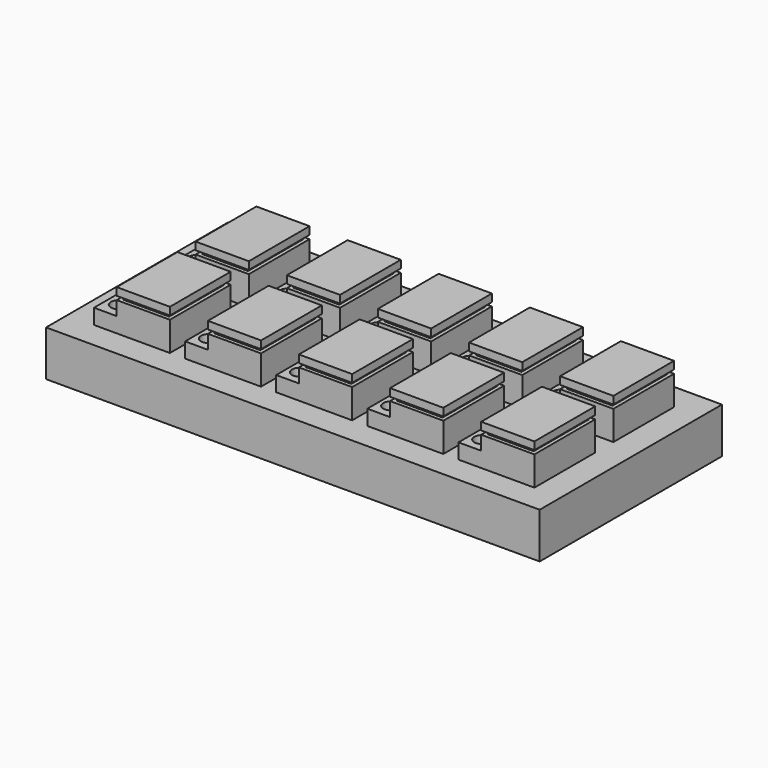
from build123d import *

# Parameters (mm, degrees)
F0_W           = 103.1875
F0_H           = 47.625
F1_DEPTH       = 9.525
F2_W           = 15.875
F2_H           = 15.875
F3_DEPTH       = 3.175
F4_W           = 11.1267840786
F4_H           = 15.875
F5_DEPTH       = 5.334
F6_W           = 11.1309718871
F6_H           = 15.875
F7_DEPTH       = 5.334
F8_W           = 11.1265123679
F8_H           = 15.875
F9_DEPTH       = 5.334
F10_W          = 11.1239126975
F10_H          = 15.875
F11_DEPTH      = 5.334
F12_W          = 11.1350612026
F12_H          = 15.875
F13_DEPTH      = 5.334
F14_W          = 11.1336731828
F14_H          = 15.875
F15_DEPTH      = 5.334
F16_W          = 11.1136997504
F16_H          = 15.875
F17_DEPTH      = 5.334
F18_W          = 11.1152978999
F18_H          = 15.875
F19_DEPTH      = 5.334
F20_W          = 11.1280665679
F20_H          = 15.875
F21_DEPTH      = 5.334
F22_W          = 11.1295790357
F22_H          = 15.875
F23_DEPTH      = 5.334
F24_W          = 11.1267840786
F24_H          = 0.7874
F25_DEPTH      = 0.7874
F26_W          = 15.0876
F26_H          = 0.7874
F27_DEPTH      = 0.7874
F28_W          = 10.3393840786
F28_H          = 0.7874
F29_DEPTH      = 0.7874
F30_W          = 14.3002
F30_H          = 0.7874
F31_DEPTH      = 0.7874
F32_W          = 15.875
F32_H          = 0.7874
F33_DEPTH      = 0.7874
F34_W          = 10.3435718871
F34_H          = 0.7874
F35_DEPTH      = 0.7874
F36_W          = 10.3435718871
F36_H          = 0.7874
F37_DEPTH      = 0.7874
F38_W          = 14.3002
F38_H          = 0.7874
F39_DEPTH      = 0.7874
F40_W          = 11.1239126975
F40_H          = 0.7648523897
F41_DEPTH      = 0.7874
F42_W          = 15.0876
F42_H          = 0.7648523897
F43_DEPTH      = 0.7874
F44_W          = 15.0876
F44_H          = 0.7648523897
F45_DEPTH      = 0.7874
F46_W          = 9.5491126975
F46_H          = 0.7648523897
F47_DEPTH      = 0.7874
F48_W          = 11.1336731828
F48_H          = 0.7874
F49_DEPTH      = 0.7874
F50_W          = 15.0876
F50_H          = 0.7874
F51_DEPTH      = 0.7874
F52_W          = 10.3462731828
F52_H          = 0.7874
F53_DEPTH      = 0.7874
F54_W          = 14.3002
F54_H          = 0.7874
F55_DEPTH      = 0.7874
F56_W          = 11.1136997504
F56_H          = 0.7874
F57_DEPTH      = 0.7874
F58_W          = 15.0876
F58_H          = 0.7874
F59_DEPTH      = 0.7874
F60_W          = 10.3262997504
F60_H          = 0.7874
F61_DEPTH      = 0.7874
F62_W          = 14.3002
F62_H          = 0.7874
F63_DEPTH      = 0.7874
F64_W          = 11.1152978999
F64_H          = 0.7874
F65_DEPTH      = 0.7874
F66_W          = 15.0876
F66_H          = 0.7874
F67_DEPTH      = 0.7874
F68_W          = 15.0876
F68_H          = 0.7874
F69_DEPTH      = 0.7874
F70_W          = 9.5404978999
F70_H          = 0.7874
F71_DEPTH      = 0.7874
F72_W          = 15.875
F72_H          = 0.7874
F73_DEPTH      = 0.7874
F74_W          = 10.3406665679
F74_H          = 0.7874
F75_DEPTH      = 0.7874
F76_W          = 10.3406665679
F76_H          = 0.7874
F77_DEPTH      = 0.7874
F78_W          = 14.3002
F78_H          = 0.7874
F79_DEPTH      = 0.7874
F80_W          = 11.1265123679
F80_H          = 0.7874
F81_DEPTH      = 0.7874
F82_W          = 15.0876
F82_H          = 0.7874
F83_DEPTH      = 0.7874
F84_W          = 15.0876
F84_H          = 0.7874
F85_DEPTH      = 0.7874
F86_W          = 9.5517123679
F86_H          = 0.7874
F87_DEPTH      = 0.7874
F88_W          = 11.1350612026
F88_H          = 0.7874
F89_DEPTH      = 0.7874
F90_W          = 15.0876
F90_H          = 0.7874
F91_DEPTH      = 0.7874
F92_W          = 15.0876
F92_H          = 0.7874
F93_DEPTH      = 0.7874
F94_W          = 9.5602612026
F94_H          = 0.7874
F95_DEPTH      = 0.7874
F96_W          = 11.1295790357
F96_H          = 0.7874
F97_DEPTH      = 0.7874
F98_W          = 15.0876
F98_H          = 0.7874
F99_DEPTH      = 0.7874
F100_W         = 10.3421790357
F100_H         = 0.7874
F101_DEPTH     = 0.7874
F102_W         = 14.3002
F102_H         = 0.7874
F103_DEPTH     = 0.7874
F104_T         = 1.905
F104_T3_DEPTH  = 19.685
F104_T5_DEPTH  = 19.685
F104_T7_DEPTH  = 19.685
F104_T9_DEPTH  = 19.685
F104_T11_DEPTH = 19.685
F104_T13_DEPTH = 19.685
F104_T15_DEPTH = 19.685
F104_T17_DEPTH = 19.685
F104_T19_DEPTH = 13.3661718871
F104_T21_DEPTH = 18.1102
F104_T23_DEPTH = 18.1102
F104_T25_DEPTH = 13.3591126975
F104_T27_DEPTH = 13.3688731828
F104_T29_DEPTH = 13.3504978999
F104_T31_DEPTH = 13.3632665679
F104_T33_DEPTH = 13.3619840786
F104_T35_DEPTH = 18.1102
F104_T37_DEPTH = 13.3617123679
F104_T39_DEPTH = 13.3702612026
F104_T41_DEPTH = 13.3488997504
F104_T43_DEPTH = 13.3647790357
F105_R         = 1.5875
F106_DEPTH     = 5.588
F107_R         = 1.5875
F108_DEPTH     = 5.588
F109_R         = 1.5875
F110_DEPTH     = 5.588
F111_R         = 1.5875
F112_DEPTH     = 5.588
F113_R         = 1.5875
F114_DEPTH     = 5.588
F115_R         = 1.5875
F116_DEPTH     = 5.588
F117_R         = 1.5875
F118_DEPTH     = 5.588
F119_R         = 1.5875
F120_DEPTH     = 5.588
F121_R         = 1.5875
F122_DEPTH     = 5.588
F123_R         = 1.5875
F124_DEPTH     = 5.588
F126_DEPTH     = 3.175


# Not quite as in the source:
# - a shell that OpenCascade refuses in one call is made with other operations: the cavity is built on its own and cut out


with BuildPart() as f1:
    # F0 (on Top) → F1 (new body)
    with BuildSketch(Plane.XY):
        with Locations((4.0335860103, -27.4054915475)):
            Rectangle(F0_W, F0_H)
    extrude(amount=F1_DEPTH)

    # F2 (on face) → F3 (join)
    with BuildSketch(Plane.XY.offset(9.525)):
        with Locations((-34.0600639897, -37.7178915475)):
            Rectangle(F2_W, F2_H)
        with Locations((-34.0600639897, -17.0930915475)):
            Rectangle(F2_W, F2_H)
        with Locations((-15.0100639897, -17.0819594264)):
            Rectangle(F2_W, F2_H)
        with Locations((-15.0100639897, -37.7178915475)):
            Rectangle(F2_W, F2_H)
        with Locations((4.0399360103, -37.7178915475)):
            Rectangle(F2_W, F2_H)
        with Locations((4.0399360103, -17.0819594264)):
            Rectangle(F2_W, F2_H)
        with Locations((23.0899360103, -17.0819594264)):
            Rectangle(F2_W, F2_H)
        with Locations((23.0899360103, -37.7178915475)):
            Rectangle(F2_W, F2_H)
        with Locations((42.1399360103, -37.7178915475)):
            Rectangle(F2_W, F2_H)
        with Locations((42.1399360103, -17.0930915475)):
            Rectangle(F2_W, F2_H)
    extrude(amount=F3_DEPTH)

    # F4 (on face) → F5 (join)
    with BuildSketch(Plane.XY.offset(12.7)):
        with Locations((44.514043971, -37.7178915475)):
            Rectangle(F4_W, F4_H)
    extrude(amount=F5_DEPTH)

    # F6 (on face) → F7 (join)
    with BuildSketch(Plane.XY.offset(12.7)):
        with Locations((44.5119500668, -17.0930915475)):
            Rectangle(F6_W, F6_H)
    extrude(amount=F7_DEPTH)

    # F8 (on face) → F9 (join)
    with BuildSketch(Plane.XY.offset(12.7)):
        with Locations((25.4641798264, -37.7178915475)):
            Rectangle(F8_W, F8_H)
    extrude(amount=F9_DEPTH)

    # F10 (on face) → F11 (join)
    with BuildSketch(Plane.XY.offset(12.7)):
        with Locations((25.4654796616, -17.0819594264)):
            Rectangle(F10_W, F10_H)
    extrude(amount=F11_DEPTH)

    # F12 (on face) → F13 (join)
    with BuildSketch(Plane.XY.offset(12.7)):
        with Locations((6.409905409, -37.7178915475)):
            Rectangle(F12_W, F12_H)
    extrude(amount=F13_DEPTH)

    # F14 (on face) → F15 (join)
    with BuildSketch(Plane.XY.offset(12.7)):
        with Locations((6.410599419, -17.0819594264)):
            Rectangle(F14_W, F14_H)
    extrude(amount=F15_DEPTH)

    # F16 (on face) → F17 (join)
    with BuildSketch(Plane.XY.offset(12.7)):
        with Locations((-12.6294138649, -37.7178915475)):
            Rectangle(F16_W, F16_H)
    extrude(amount=F17_DEPTH)

    # F18 (on face) → F19 (join)
    with BuildSketch(Plane.XY.offset(12.7)):
        with Locations((-12.6302129396, -17.0819594264)):
            Rectangle(F18_W, F18_H)
    extrude(amount=F19_DEPTH)

    # F20 (on face) → F21 (join)
    with BuildSketch(Plane.XY.offset(12.7)):
        with Locations((-31.6865972736, -17.0930915475)):
            Rectangle(F20_W, F20_H)
    extrude(amount=F21_DEPTH)

    # F22 (on face) → F23 (join)
    with BuildSketch(Plane.XY.offset(12.7)):
        with Locations((-31.6873535075, -37.7178915475)):
            Rectangle(F22_W, F22_H)
    extrude(amount=F23_DEPTH)

    # F24 (on face) → F25 (cut)
    with BuildSketch(Plane.XZ.offset(45.6553915475)):
        with Locations((44.514043971, 16.0401)):
            Rectangle(F24_W, F24_H)
    extrude(amount=-F25_DEPTH, mode=Mode.SUBTRACT)

    # F26 (on face) → F27 (cut)
    with BuildSketch(Plane.YZ.offset(50.0774360103)):
        with Locations((-37.3241915475, 16.0401)):
            Rectangle(F26_W, F26_H)
    extrude(amount=-F27_DEPTH, mode=Mode.SUBTRACT)

    # F28 (on face) → F29 (cut)
    with BuildSketch(Plane(origin=(0, -29.7803915475, 0), x_dir=(-1, 0, 0), z_dir=(0, 1, 0))):
        with Locations((-44.120343971, 16.0401)):
            Rectangle(F28_W, F28_H)
    extrude(amount=-F29_DEPTH, mode=Mode.SUBTRACT)

    # F30 (on face) → F31 (cut)
    with BuildSketch(Plane(origin=(38.9506519317, 0, 0), x_dir=(0, -1, 0), z_dir=(-1, 0, 0))):
        with Locations((37.7178915475, 16.0401)):
            Rectangle(F30_W, F30_H)
    extrude(amount=-F31_DEPTH, mode=Mode.SUBTRACT)

    # F32 (on face) → F33 (cut)
    with BuildSketch(Plane.YZ.offset(50.0774360103)):
        with Locations((-17.0930915475, 16.0401)):
            Rectangle(F32_W, F32_H)
    extrude(amount=-F33_DEPTH, mode=Mode.SUBTRACT)

    # F34 (on face) → F35 (cut)
    with BuildSketch(Plane(origin=(0, -9.1555915475, 0), x_dir=(-1, 0, 0), z_dir=(0, 1, 0))):
        with Locations((-44.1182500668, 16.0401)):
            Rectangle(F34_W, F34_H)
    extrude(amount=-F35_DEPTH, mode=Mode.SUBTRACT)

    # F36 (on face) → F37 (cut)
    with BuildSketch(Plane.XZ.offset(25.0305915475)):
        with Locations((44.1182500668, 16.0401)):
            Rectangle(F36_W, F36_H)
    extrude(amount=-F37_DEPTH, mode=Mode.SUBTRACT)

    # F38 (on face) → F39 (cut)
    with BuildSketch(Plane(origin=(38.9464641232, 0, 0), x_dir=(0, -1, 0), z_dir=(-1, 0, 0))):
        with Locations((17.0930915475, 16.0401)):
            Rectangle(F38_W, F38_H)
    extrude(amount=-F39_DEPTH, mode=Mode.SUBTRACT)

    # F40 (on face) → F41 (cut)
    with BuildSketch(Plane(origin=(0, -9.1444594264, 0), x_dir=(-1, 0, 0), z_dir=(0, 1, 0))):
        with Locations((-25.4654796616, 16.0446381196)):
            Rectangle(F40_W, F40_H)
    extrude(amount=-F41_DEPTH, mode=Mode.SUBTRACT)

    # F42 (on face) → F43 (cut)
    with BuildSketch(Plane.YZ.offset(31.0274360103)):
        with Locations((-17.4756594264, 16.0446381196)):
            Rectangle(F42_W, F42_H)
    extrude(amount=-F43_DEPTH, mode=Mode.SUBTRACT)

    # F44 (on face) → F45 (cut)
    with BuildSketch(Plane(origin=(19.9035233129, 0, 0), x_dir=(0, -1, 0), z_dir=(-1, 0, 0))):
        with Locations((17.4756594264, 16.0446381196)):
            Rectangle(F44_W, F44_H)
    extrude(amount=-F45_DEPTH, mode=Mode.SUBTRACT)

    # F46 (on face) → F47 (cut)
    with BuildSketch(Plane.XZ.offset(25.0194594264)):
        with Locations((25.4654796616, 16.0446381196)):
            Rectangle(F46_W, F46_H)
    extrude(amount=-F47_DEPTH, mode=Mode.SUBTRACT)

    # F48 (on face) → F49 (cut)
    with BuildSketch(Plane(origin=(0, -9.1444594264, 0), x_dir=(-1, 0, 0), z_dir=(0, 1, 0))):
        with Locations((-6.410599419, 16.0401)):
            Rectangle(F48_W, F48_H)
    extrude(amount=-F49_DEPTH, mode=Mode.SUBTRACT)

    # F50 (on face) → F51 (cut)
    with BuildSketch(Plane(origin=(0.8437628276, 0, 0), x_dir=(0, -1, 0), z_dir=(-1, 0, 0))):
        with Locations((17.4756594264, 16.0401)):
            Rectangle(F50_W, F50_H)
    extrude(amount=-F51_DEPTH, mode=Mode.SUBTRACT)

    # F52 (on face) → F53 (cut)
    with BuildSketch(Plane.XZ.offset(25.0194594264)):
        with Locations((6.804299419, 16.0401)):
            Rectangle(F52_W, F52_H)
    extrude(amount=-F53_DEPTH, mode=Mode.SUBTRACT)

    # F54 (on face) → F55 (cut)
    with BuildSketch(Plane.YZ.offset(11.9774360103)):
        with Locations((-17.0819594264, 16.0401)):
            Rectangle(F54_W, F54_H)
    extrude(amount=-F55_DEPTH, mode=Mode.SUBTRACT)

    # F56 (on face) → F57 (cut)
    with BuildSketch(Plane.XZ.offset(45.6553915475)):
        with Locations((-12.6294138649, 16.0401)):
            Rectangle(F56_W, F56_H)
    extrude(amount=-F57_DEPTH, mode=Mode.SUBTRACT)

    # F58 (on face) → F59 (cut)
    with BuildSketch(Plane(origin=(-18.1862637401, 0, 0), x_dir=(0, -1, 0), z_dir=(-1, 0, 0))):
        with Locations((37.3241915475, 16.0401)):
            Rectangle(F58_W, F58_H)
    extrude(amount=-F59_DEPTH, mode=Mode.SUBTRACT)

    # F60 (on face) → F61 (cut)
    with BuildSketch(Plane(origin=(0, -29.7803915475, 0), x_dir=(-1, 0, 0), z_dir=(0, 1, 0))):
        with Locations((12.2357138649, 16.0401)):
            Rectangle(F60_W, F60_H)
    extrude(amount=-F61_DEPTH, mode=Mode.SUBTRACT)

    # F62 (on face) → F63 (cut)
    with BuildSketch(Plane.YZ.offset(-7.0725639897)):
        with Locations((-37.7178915475, 16.0401)):
            Rectangle(F62_W, F62_H)
    extrude(amount=-F63_DEPTH, mode=Mode.SUBTRACT)

    # F64 (on face) → F65 (cut)
    with BuildSketch(Plane(origin=(0, -9.1444594264, 0), x_dir=(-1, 0, 0), z_dir=(0, 1, 0))):
        with Locations((12.6302129396, 16.0401)):
            Rectangle(F64_W, F64_H)
    extrude(amount=-F65_DEPTH, mode=Mode.SUBTRACT)

    # F66 (on face) → F67 (cut)
    with BuildSketch(Plane.YZ.offset(-7.0725639897)):
        with Locations((-17.4756594264, 16.0401)):
            Rectangle(F66_W, F66_H)
    extrude(amount=-F67_DEPTH, mode=Mode.SUBTRACT)

    # F68 (on face) → F69 (cut)
    with BuildSketch(Plane(origin=(-18.1878618896, 0, 0), x_dir=(0, -1, 0), z_dir=(-1, 0, 0))):
        with Locations((17.4756594264, 16.0401)):
            Rectangle(F68_W, F68_H)
    extrude(amount=-F69_DEPTH, mode=Mode.SUBTRACT)

    # F70 (on face) → F71 (cut)
    with BuildSketch(Plane.XZ.offset(25.0194594264)):
        with Locations((-12.6302129396, 16.0401)):
            Rectangle(F70_W, F70_H)
    extrude(amount=-F71_DEPTH, mode=Mode.SUBTRACT)

    # F72 (on face) → F73 (cut)
    with BuildSketch(Plane.YZ.offset(-26.1225639897)):
        with Locations((-17.0930915475, 16.0401)):
            Rectangle(F72_W, F72_H)
    extrude(amount=-F73_DEPTH, mode=Mode.SUBTRACT)

    # F74 (on face) → F75 (cut)
    with BuildSketch(Plane.XZ.offset(25.0305915475)):
        with Locations((-32.0802972736, 16.0401)):
            Rectangle(F74_W, F74_H)
    extrude(amount=-F75_DEPTH, mode=Mode.SUBTRACT)

    # F76 (on face) → F77 (cut)
    with BuildSketch(Plane(origin=(0, -9.1555915475, 0), x_dir=(-1, 0, 0), z_dir=(0, 1, 0))):
        with Locations((32.0802972736, 16.0401)):
            Rectangle(F76_W, F76_H)
    extrude(amount=-F77_DEPTH, mode=Mode.SUBTRACT)

    # F78 (on face) → F79 (cut)
    with BuildSketch(Plane(origin=(-37.2506305575, 0, 0), x_dir=(0, -1, 0), z_dir=(-1, 0, 0))):
        with Locations((17.0930915475, 16.0401)):
            Rectangle(F78_W, F78_H)
    extrude(amount=-F79_DEPTH, mode=Mode.SUBTRACT)

    # F80 (on face) → F81 (cut)
    with BuildSketch(Plane.XZ.offset(45.6553915475)):
        with Locations((25.4641798264, 16.0401)):
            Rectangle(F80_W, F80_H)
    extrude(amount=-F81_DEPTH, mode=Mode.SUBTRACT)

    # F82 (on face) → F83 (cut)
    with BuildSketch(Plane.YZ.offset(31.0274360103)):
        with Locations((-37.3241915475, 16.0401)):
            Rectangle(F82_W, F82_H)
    extrude(amount=-F83_DEPTH, mode=Mode.SUBTRACT)

    # F84 (on face) → F85 (cut)
    with BuildSketch(Plane(origin=(19.9009236425, 0, 0), x_dir=(0, -1, 0), z_dir=(-1, 0, 0))):
        with Locations((37.3241915475, 16.0401)):
            Rectangle(F84_W, F84_H)
    extrude(amount=-F85_DEPTH, mode=Mode.SUBTRACT)

    # F86 (on face) → F87 (cut)
    with BuildSketch(Plane(origin=(0, -29.7803915475, 0), x_dir=(-1, 0, 0), z_dir=(0, 1, 0))):
        with Locations((-25.4641798264, 16.0401)):
            Rectangle(F86_W, F86_H)
    extrude(amount=-F87_DEPTH, mode=Mode.SUBTRACT)

    # F88 (on face) → F89 (cut)
    with BuildSketch(Plane.XZ.offset(45.6553915475)):
        with Locations((6.409905409, 16.0401)):
            Rectangle(F88_W, F88_H)
    extrude(amount=-F89_DEPTH, mode=Mode.SUBTRACT)

    # F90 (on face) → F91 (cut)
    with BuildSketch(Plane(origin=(0.8423748077, 0, 0), x_dir=(0, -1, 0), z_dir=(-1, 0, 0))):
        with Locations((37.3241915475, 16.0401)):
            Rectangle(F90_W, F90_H)
    extrude(amount=-F91_DEPTH, mode=Mode.SUBTRACT)

    # F92 (on face) → F93 (cut)
    with BuildSketch(Plane.YZ.offset(11.9774360103)):
        with Locations((-37.3241915475, 16.0401)):
            Rectangle(F92_W, F92_H)
    extrude(amount=-F93_DEPTH, mode=Mode.SUBTRACT)

    # F94 (on face) → F95 (cut)
    with BuildSketch(Plane(origin=(0, -29.7803915475, 0), x_dir=(-1, 0, 0), z_dir=(0, 1, 0))):
        with Locations((-6.409905409, 16.0401)):
            Rectangle(F94_W, F94_H)
    extrude(amount=-F95_DEPTH, mode=Mode.SUBTRACT)

    # F96 (on face) → F97 (cut)
    with BuildSketch(Plane.XZ.offset(45.6553915475)):
        with Locations((-31.6873535075, 16.0401)):
            Rectangle(F96_W, F96_H)
    extrude(amount=-F97_DEPTH, mode=Mode.SUBTRACT)

    # F98 (on face) → F99 (cut)
    with BuildSketch(Plane(origin=(-37.2521430254, 0, 0), x_dir=(0, -1, 0), z_dir=(-1, 0, 0))):
        with Locations((37.3241915475, 16.0401)):
            Rectangle(F98_W, F98_H)
    extrude(amount=-F99_DEPTH, mode=Mode.SUBTRACT)

    # F100 (on face) → F101 (cut)
    with BuildSketch(Plane(origin=(0, -29.7803915475, 0), x_dir=(-1, 0, 0), z_dir=(0, 1, 0))):
        with Locations((31.2936535075, 16.0401)):
            Rectangle(F100_W, F100_H)
    extrude(amount=-F101_DEPTH, mode=Mode.SUBTRACT)

    # F102 (on face) → F103 (cut)
    with BuildSketch(Plane.YZ.offset(-26.1225639897)):
        with Locations((-37.7178915475, 16.0401)):
            Rectangle(F102_W, F102_H)
    extrude(amount=-F103_DEPTH, mode=Mode.SUBTRACT)

    # F104: shell of thickness 1.905, made by hand


with BuildPart() as f104_core1:
    # F104_t2: copy of F1
    add(f1.part)

    # the walls: a layer under each face that stays
    f104_faces = [f104_core1.faces().sort_by_distance(p)[0] for p in [
        (4.0335860103, -3.5929915475, 4.7625),
        (4.0335860103, -27.4054915475, 9.525),
        (42.1399360103, -9.1555915475, 12.5857),
        (36.5744500668, -17.0930915475, 12.7),
        (38.9464641232, -17.0930915475, 14.1732),
        (39.3174965194, -24.5014248808, 15.6464),
        (39.7338641232, -17.0930915475, 16.0401),
        (49.7064036141, -9.6847582141, 16.4338),
        (44.5119500668, -9.1555915475, 17.2339),
        (44.5119500668, -17.0930915475, 18.034),
        (50.0774360103, -17.0930915475, 17.2339),
        (44.5119500668, -25.0305915475, 17.2339),
        (38.9464641232, -17.0930915475, 17.2339),
        (44.5119500668, -9.9429915475, 16.0401),
        (49.2900360103, -17.0930915475, 16.0401),
        (44.5119500668, -24.2431915475, 16.0401),
        (50.0774360103, -17.0930915475, 12.5857),
        (42.1399360103, -25.0305915475, 12.5857),
        (34.2024360103, -17.0930915475, 11.1125),
        (23.0899360103, -9.1444594264, 12.5936059624),
        (20.2743204028, -24.4902927597, 15.6622119248),
        (25.4654796616, -24.2320594264, 16.0446381196),
        (20.2743204028, -9.6736260931, 16.4270643145),
        (19.9035233129, -17.0819594264, 17.2305321572),
        (25.4654796616, -17.0819594264, 18.034),
        (25.4654796616, -9.1444594264, 17.2305321572),
        (31.0274360103, -17.0819594264, 17.2305321572),
        (25.4654796616, -25.0194594264, 17.2305321572),
        (20.6909233129, -17.0819594264, 16.0446381196),
        (25.4654796616, -9.9318594264, 16.0446381196),
        (30.2400360103, -17.0819594264, 16.0446381196),
        (19.9035233129, -17.0819594264, 14.1811059624),
        (17.5279796616, -17.0819594264, 12.7),
        (31.0274360103, -17.0819594264, 12.5936059624),
        (23.0899360103, -25.0194594264, 12.5936059624),
        (15.1524360103, -17.0819594264, 11.1125),
        (4.0399360103, -9.1444594264, 12.5857),
        (1.214885267, -9.6736260931, 15.6464),
        (11.1900360103, -17.0819594264, 16.0401),
        (11.6063135709, -24.4902927597, 16.4338),
        (0.8437628276, -17.0819594264, 17.2339),
        (6.410599419, -17.0819594264, 18.034),
        (6.410599419, -9.1444594264, 17.2339),
        (11.9774360103, -17.0819594264, 17.2339),
        (6.410599419, -25.0194594264, 17.2339),
        (6.410599419, -24.2320594264, 16.0401),
        (1.6311628276, -17.0819594264, 16.0401),
        (6.410599419, -9.9318594264, 16.0401),
        (0.8437628276, -17.0819594264, 14.1732),
        (-1.526900581, -17.0819594264, 12.7),
        (11.9774360103, -17.0819594264, 12.5857),
        (4.0399360103, -25.0194594264, 12.5857),
        (-3.8975639897, -17.0819594264, 11.1125),
        (-7.0725639897, -17.0819594264, 12.5857),
        (-7.4430739197, -24.4902927597, 15.6464),
        (-12.6302129396, -24.2320594264, 16.0401),
        (-17.8173519596, -9.6736260931, 16.4338),
        (-18.1878618896, -17.0819594264, 17.2339),
        (-12.6302129396, -17.0819594264, 18.034),
        (-12.6302129396, -9.1444594264, 17.2339),
        (-7.0725639897, -17.0819594264, 17.2339),
        (-12.6302129396, -25.0194594264, 17.2339),
        (-17.4004618896, -17.0819594264, 16.0401),
        (-12.6302129396, -9.9318594264, 16.0401),
        (-7.8599639897, -17.0819594264, 16.0401),
        (-18.1878618896, -17.0819594264, 14.1732),
        (-20.5677129396, -17.0819594264, 12.7),
        (-15.0100639897, -25.0194594264, 12.5857),
        (-22.9475639897, -17.0819594264, 11.1125),
        (-15.0100639897, -9.1444594264, 12.5857),
        (-34.0600639897, -25.0305915475, 12.5857),
        (-36.8796950053, -24.5014248808, 15.6464),
        (-36.4632305575, -17.0930915475, 16.0401),
        (-36.8796950053, -9.6847582141, 16.4338),
        (-26.1225639897, -17.0930915475, 17.2339),
        (-31.6865972736, -17.0930915475, 18.034),
        (-31.6865972736, -25.0305915475, 17.2339),
        (-37.2506305575, -17.0930915475, 17.2339),
        (-31.6865972736, -9.1555915475, 17.2339),
        (-31.6865972736, -9.9429915475, 16.0401),
        (-26.9099639897, -17.0930915475, 16.0401),
        (-31.6865972736, -24.2431915475, 16.0401),
        (-37.2506305575, -17.0930915475, 14.1732),
        (-39.6240972736, -17.0930915475, 12.7),
        (-41.9975639897, -17.0930915475, 11.1125),
        (-34.0600639897, -9.1555915475, 12.5857),
        (-26.1225639897, -17.0930915475, 12.5857),
        (34.2024360103, -37.7178915475, 11.1125),
        (36.576543971, -37.7178915475, 12.7),
        (38.9506519317, -37.7178915475, 14.1732),
        (39.3215447344, -30.3095582141, 15.6464),
        (39.7380519317, -37.7178915475, 16.0401),
        (39.3215447344, -30.3095582141, 16.4338),
        (50.0774360103, -37.7178915475, 17.2339),
        (44.514043971, -37.7178915475, 18.034),
        (44.514043971, -45.6553915475, 17.2339),
        (38.9506519317, -37.7178915475, 17.2339),
        (44.514043971, -29.7803915475, 17.2339),
        (44.514043971, -30.5677915475, 16.0401),
        (49.2900360103, -37.7178915475, 16.0401),
        (44.514043971, -44.8679915475, 16.0401),
        (42.1399360103, -29.7803915475, 12.5857),
        (50.0774360103, -37.7178915475, 12.5857),
        (42.1399360103, -45.6553915475, 12.5857),
        (23.0899360103, -29.7803915475, 12.5857),
        (17.5266798264, -37.7178915475, 12.7),
        (19.9009236425, -37.7178915475, 14.1732),
        (20.2718073881, -30.3095582141, 15.6464),
        (25.4641798264, -30.5677915475, 16.0401),
        (30.6565522647, -45.1262248808, 16.4338),
        (31.0274360103, -37.7178915475, 17.2339),
        (25.4641798264, -37.7178915475, 18.034),
        (25.4641798264, -45.6553915475, 17.2339),
        (19.9009236425, -37.7178915475, 17.2339),
        (25.4641798264, -29.7803915475, 17.2339),
        (30.2400360103, -37.7178915475, 16.0401),
        (25.4641798264, -44.8679915475, 16.0401),
        (20.6883236425, -37.7178915475, 16.0401),
        (31.0274360103, -37.7178915475, 12.5857),
        (23.0899360103, -45.6553915475, 12.5857),
        (15.1524360103, -37.7178915475, 11.1125),
        (4.0399360103, -45.6553915475, 12.5857),
        (-1.527594591, -37.7178915475, 12.7),
        (0.8423748077, -37.7178915475, 14.1732),
        (1.2135435144, -30.3095582141, 15.6464),
        (6.409905409, -30.5677915475, 16.0401),
        (11.6062673036, -30.3095582141, 16.4338),
        (6.409905409, -45.6553915475, 17.2339),
        (6.409905409, -37.7178915475, 18.034),
        (0.8423748077, -37.7178915475, 17.2339),
        (6.409905409, -29.7803915475, 17.2339),
        (11.9774360103, -37.7178915475, 17.2339),
        (11.1900360103, -37.7178915475, 16.0401),
        (6.409905409, -44.8679915475, 16.0401),
        (1.6297748077, -37.7178915475, 16.0401),
        (-3.8975639897, -37.7178915475, 11.1125),
        (4.0399360103, -29.7803915475, 12.5857),
        (11.9774360103, -37.7178915475, 12.5857),
        (-7.0725639897, -37.7178915475, 12.5857),
        (-7.443020648, -30.3095582141, 15.6464),
        (-7.8599639897, -37.7178915475, 16.0401),
        (-17.8158070817, -45.1262248808, 16.4338),
        (-12.6294138649, -45.6553915475, 17.2339),
        (-12.6294138649, -37.7178915475, 18.034),
        (-18.1862637401, -37.7178915475, 17.2339),
        (-12.6294138649, -29.7803915475, 17.2339),
        (-7.0725639897, -37.7178915475, 17.2339),
        (-12.6294138649, -44.8679915475, 16.0401),
        (-17.3988637401, -37.7178915475, 16.0401),
        (-12.6294138649, -30.5677915475, 16.0401),
        (-18.1862637401, -37.7178915475, 14.1732),
        (-20.5669138649, -37.7178915475, 12.7),
        (-15.0100639897, -45.6553915475, 12.5857),
        (-22.9475639897, -37.7178915475, 11.1125),
        (-15.0100639897, -29.7803915475, 12.5857),
        (-34.0600639897, -29.7803915475, 12.5857),
        (-39.6248535075, -37.7178915475, 12.7),
        (-37.2521430254, -37.7178915475, 14.1732),
        (-36.8811570575, -30.3095582141, 15.6464),
        (-26.9099639897, -37.7178915475, 16.0401),
        (-36.8811570575, -45.1262248808, 16.4338),
        (-31.6873535075, -45.6553915475, 17.2339),
        (-31.6873535075, -37.7178915475, 18.034),
        (-37.2521430254, -37.7178915475, 17.2339),
        (-31.6873535075, -29.7803915475, 17.2339),
        (-26.1225639897, -37.7178915475, 17.2339),
        (-31.6873535075, -44.8679915475, 16.0401),
        (-36.4647430254, -37.7178915475, 16.0401),
        (-31.6873535075, -30.5677915475, 16.0401),
        (-26.1225639897, -37.7178915475, 12.5857),
        (-34.0600639897, -45.6553915475, 12.5857),
        (-41.9975639897, -37.7178915475, 11.1125),
        (4.0335860103, -51.2179915475, 4.7625),
        (-47.5601639897, -27.4054915475, 4.7625),
        (55.6273360103, -27.4054915475, 4.7625),
    ]]
    thicken(f104_faces, amount=-F104_T, mode=Mode.SUBTRACT)

    # F104_s4 → F104_t3 (cut)
    with BuildSketch(Plane.XZ.offset(27.8753915475)):
        Polygon((-42.0166139897, 9.54405), (-41.9975639897, 7.62), (-40.0925639897, 7.62), (-40.0925639897, 9.525), align=None)
        Polygon((-26.1035139897, 9.54405), (-26.1225639897, 7.62), (-28.0275639897, 7.62), (-28.0275639897, 9.525), align=None)
        Polygon((-22.9666139897, 9.54405), (-22.9475639897, 7.62), (-21.0425639897, 7.62), (-21.0425639897, 9.525), align=None)
        Polygon((-7.0535139897, 9.54405), (-7.0725639897, 7.62), (-8.9775639897, 7.62), (-8.9775639897, 9.525), align=None)
        Polygon((11.9964860103, 9.54405), (11.9774360103, 7.62), (10.0724360103, 7.62), (10.0724360103, 9.525), align=None)
        Polygon((-3.9166139897, 9.54405), (-3.8975639897, 7.62), (-1.9925639897, 7.62), (-1.9925639897, 9.525), align=None)
        Polygon((15.1333860103, 9.54405), (15.1524360103, 7.62), (17.0574360103, 7.62), (17.0574360103, 9.525), align=None)
        Polygon((31.0464860103, 9.54405), (31.0274360103, 7.62), (29.1224360103, 7.62), (29.1224360103, 9.525), align=None)
        Polygon((50.0964860103, 9.54405), (50.0774360103, 7.62), (48.1724360103, 7.62), (48.1724360103, 9.525), align=None)
        Polygon((34.1833860103, 9.54405), (34.2024360103, 7.62), (36.1074360103, 7.62), (36.1074360103, 9.525), align=None)
        Polygon((38.9316019317, 12.71905), (38.9506519317, 10.795), (40.8556519317, 10.795), (40.8556519317, 12.7), align=None)
        Polygon((19.8818736425, 12.71905), (19.9009236425, 10.795), (21.8059236425, 10.795), (21.8059236425, 12.7), align=None)
        Polygon((0.8233248077, 12.71905), (0.8423748077, 10.795), (2.7473748077, 10.795), (2.7473748077, 12.7), align=None)
        Polygon((-18.2053137401, 12.71905), (-16.2812637401, 12.7), (-16.2812637401, 10.795), (-18.1862637401, 10.795), align=None)
        Polygon((-37.2711930254, 12.71905), (-37.2521430254, 10.795), (-35.3471430254, 10.795), (-35.3471430254, 12.7), align=None)
    extrude(amount=F104_T3_DEPTH, mode=Mode.SUBTRACT)

    # F104_s6 → F104_t5 (cut)
    with BuildSketch(Plane.YZ.offset(-43.9025639897)):
        Polygon((-45.6744415475, 9.54405), (-45.6553915475, 7.62), (-43.7503915475, 7.62), (-43.7503915475, 9.525), align=None)
        Polygon((-29.7613415475, 9.54405), (-29.7803915475, 7.62), (-31.6853915475, 7.62), (-31.6853915475, 9.525), align=None)
        Polygon((-9.1365415475, 9.54405), (-9.1555915475, 7.62), (-11.0605915475, 7.62), (-11.0605915475, 9.525), align=None)
        Polygon((-25.0496415475, 9.54405), (-25.0305915475, 7.62), (-23.1255915475, 7.62), (-23.1255915475, 9.525), align=None)
    extrude(amount=F104_T5_DEPTH, mode=Mode.SUBTRACT)

    # F104_s8 → F104_t7 (cut)
    with BuildSketch(Plane.YZ.offset(-24.8525639897)):
        Polygon((-29.7613415475, 9.54405), (-29.7803915475, 7.62), (-31.6853915475, 7.62), (-31.6853915475, 9.525), align=None)
        Polygon((-45.6744415475, 9.54405), (-45.6553915475, 7.62), (-43.7503915475, 7.62), (-43.7503915475, 9.525), align=None)
        Polygon((-9.1254094264, 9.54405), (-9.1444594264, 7.62), (-11.0494594264, 7.62), (-11.0494594264, 9.525), align=None)
        Polygon((-25.0385094264, 9.54405), (-25.0194594264, 7.62), (-23.1144594264, 7.62), (-23.1144594264, 9.525), align=None)
    extrude(amount=F104_T7_DEPTH, mode=Mode.SUBTRACT)

    # F104_s10 → F104_t9 (cut)
    with BuildSketch(Plane.YZ.offset(-5.8025639897)):
        Polygon((-29.7613415475, 9.54405), (-29.7803915475, 7.62), (-31.6853915475, 7.62), (-31.6853915475, 9.525), align=None)
        Polygon((-45.6744415475, 9.54405), (-45.6553915475, 7.62), (-43.7503915475, 7.62), (-43.7503915475, 9.525), align=None)
        Polygon((-25.0385094264, 9.54405), (-25.0194594264, 7.62), (-23.1144594264, 7.62), (-23.1144594264, 9.525), align=None)
        Polygon((-9.1254094264, 9.54405), (-9.1444594264, 7.62), (-11.0494594264, 7.62), (-11.0494594264, 9.525), align=None)
    extrude(amount=F104_T9_DEPTH, mode=Mode.SUBTRACT)

    # F104_s12 → F104_t11 (cut)
    with BuildSketch(Plane.YZ.offset(13.2474360103)):
        Polygon((-45.6744415475, 9.54405), (-45.6553915475, 7.62), (-43.7503915475, 7.62), (-43.7503915475, 9.525), align=None)
        Polygon((-29.7613415475, 9.54405), (-29.7803915475, 7.62), (-31.6853915475, 7.62), (-31.6853915475, 9.525), align=None)
        Polygon((-25.0385094264, 9.54405), (-25.0194594264, 7.62), (-23.1144594264, 7.62), (-23.1144594264, 9.525), align=None)
        Polygon((-9.1254094264, 9.54405), (-9.1444594264, 7.62), (-11.0494594264, 7.62), (-11.0494594264, 9.525), align=None)
    extrude(amount=F104_T11_DEPTH, mode=Mode.SUBTRACT)

    # F104_s14 → F104_t13 (cut)
    with BuildSketch(Plane.YZ.offset(32.2974360103)):
        Polygon((-45.6744415475, 9.54405), (-45.6553915475, 7.62), (-43.7503915475, 7.62), (-43.7503915475, 9.525), align=None)
        Polygon((-29.7613415475, 9.54405), (-29.7803915475, 7.62), (-31.6853915475, 7.62), (-31.6853915475, 9.525), align=None)
        Polygon((-25.0496415475, 9.54405), (-25.0305915475, 7.62), (-23.1255915475, 7.62), (-23.1255915475, 9.525), align=None)
        Polygon((-9.1365415475, 9.54405), (-9.1555915475, 7.62), (-11.0605915475, 7.62), (-11.0605915475, 9.525), align=None)
    extrude(amount=F104_T13_DEPTH, mode=Mode.SUBTRACT)

    # F104_s16 → F104_t15 (cut)
    with BuildSketch(Plane.XZ.offset(7.2505915475)):
        Polygon((-26.1035139897, 9.54405), (-26.1225639897, 7.62), (-28.0275639897, 7.62), (-28.0275639897, 9.525), align=None)
        Polygon((-42.0166139897, 9.54405), (-41.9975639897, 7.62), (-40.0925639897, 7.62), (-40.0925639897, 9.525), align=None)
        Polygon((34.1833860103, 9.54405), (34.2024360103, 7.62), (36.1074360103, 7.62), (36.1074360103, 9.525), align=None)
        Polygon((50.0964860103, 9.54405), (50.0774360103, 7.62), (48.1724360103, 7.62), (48.1724360103, 9.525), align=None)
        Polygon((38.9274141232, 12.71905), (38.9464641232, 10.795), (40.8514641232, 10.795), (40.8514641232, 12.7), align=None)
        Polygon((-37.2696805575, 12.71905), (-35.3456305575, 12.7), (-35.3456305575, 10.795), (-37.2506305575, 10.795), align=None)
    extrude(amount=F104_T15_DEPTH, mode=Mode.SUBTRACT)

    # F104_s18 → F104_t17 (cut)
    with BuildSketch(Plane.XZ.offset(7.2394594264)):
        Polygon((-22.9666139897, 9.54405), (-22.9475639897, 7.62), (-21.0425639897, 7.62), (-21.0425639897, 9.525), align=None)
        Polygon((-7.0535139897, 9.54405), (-7.0725639897, 7.62), (-8.9775639897, 7.62), (-8.9775639897, 9.525), align=None)
        Polygon((-3.9166139897, 9.54405), (-3.8975639897, 7.62), (-1.9925639897, 7.62), (-1.9925639897, 9.525), align=None)
        Polygon((11.9964860103, 9.54405), (11.9774360103, 7.62), (10.0724360103, 7.62), (10.0724360103, 9.525), align=None)
        Polygon((15.1333860103, 9.54405), (15.1524360103, 7.62), (17.0574360103, 7.62), (17.0574360103, 9.525), align=None)
        Polygon((31.0464860103, 9.54405), (31.0274360103, 7.62), (29.1224360103, 7.62), (29.1224360103, 9.525), align=None)
        Polygon((19.8844733129, 12.71905), (21.8085233129, 12.7), (21.8085233129, 10.795), (19.9035233129, 10.795), align=None)
        Polygon((0.8247128276, 12.71905), (2.7487628276, 12.7), (2.7487628276, 10.795), (0.8437628276, 10.795), align=None)
        Polygon((-18.2069118896, 12.71905), (-16.2828618896, 12.7), (-16.2828618896, 10.795), (-18.1878618896, 10.795), align=None)
    extrude(amount=F104_T17_DEPTH, mode=Mode.SUBTRACT)

    # F104_s20 → F104_t19 (cut)
    with BuildSketch(Plane.YZ.offset(37.8288641232)):
        Polygon((-24.2622415475, 15.66545), (-24.2431915475, 13.7414), (-22.3381915475, 13.7414), (-22.3381915475, 15.6464), align=None)
        Polygon((-9.9239415475, 15.66545), (-9.9429915475, 13.7414), (-11.8479915475, 13.7414), (-11.8479915475, 15.6464), align=None)
        Polygon((-9.9239415475, 16.41475), (-9.9429915475, 18.3388), (-11.8479915475, 18.3388), (-11.8479915475, 16.4338), align=None)
        Polygon((-24.2622415475, 16.41475), (-24.2431915475, 18.3388), (-22.3381915475, 18.3388), (-22.3381915475, 16.4338), align=None)
    extrude(amount=F104_T19_DEPTH, mode=Mode.SUBTRACT)

    # F104_s22 → F104_t21 (cut)
    with BuildSketch(Plane.XZ.offset(8.0379915475)):
        Polygon((49.3090860103, 15.66545), (49.2900360103, 13.7414), (47.3850360103, 13.7414), (47.3850360103, 15.6464), align=None)
        Polygon((39.7148141232, 15.66545), (39.7338641232, 13.7414), (41.6388641232, 13.7414), (41.6388641232, 15.6464), align=None)
        Polygon((39.7148141232, 16.41475), (41.6388641232, 16.4338), (41.6388641232, 18.3388), (39.7338641232, 18.3388), align=None)
        Polygon((49.3090860103, 16.41475), (49.2900360103, 18.3388), (47.3850360103, 18.3388), (47.3850360103, 16.4338), align=None)
        Polygon((-26.8909139897, 15.66545), (-26.9099639897, 13.7414), (-28.8149639897, 13.7414), (-28.8149639897, 15.6464), align=None)
        Polygon((-36.4822805575, 15.66545), (-36.4632305575, 13.7414), (-34.5582305575, 13.7414), (-34.5582305575, 15.6464), align=None)
        Polygon((-36.4822805575, 16.41475), (-34.5582305575, 16.4338), (-34.5582305575, 18.3388), (-36.4632305575, 18.3388), align=None)
        Polygon((-26.8909139897, 16.41475), (-26.9099639897, 18.3388), (-28.8149639897, 18.3388), (-28.8149639897, 16.4338), align=None)
    extrude(amount=F104_T21_DEPTH, mode=Mode.SUBTRACT)

    # F104_s24 → F104_t23 (cut)
    with BuildSketch(Plane.XZ.offset(8.0268594264)):
        Polygon((30.2590860103, 15.6812619248), (30.2400360103, 13.7572119248), (28.3350360103, 13.7572119248), (28.3350360103, 15.6622119248), align=None)
        Polygon((20.6718733129, 15.6812619248), (20.6909233129, 13.7572119248), (22.5959233129, 13.7572119248), (22.5959233129, 15.6622119248), align=None)
        Polygon((20.6718733129, 16.4080143145), (20.6909233129, 18.3320643145), (22.5959233129, 18.3320643145), (22.5959233129, 16.4270643145), align=None)
        Polygon((30.2590860103, 16.4080143145), (30.2400360103, 18.3320643145), (28.3350360103, 18.3320643145), (28.3350360103, 16.4270643145), align=None)
        Polygon((1.6121128276, 15.66545), (1.6311628276, 13.7414), (3.5361628276, 13.7414), (3.5361628276, 15.6464), align=None)
        Polygon((11.2090860103, 15.66545), (11.1900360103, 13.7414), (9.2850360103, 13.7414), (9.2850360103, 15.6464), align=None)
        Polygon((11.2090860103, 16.41475), (9.2850360103, 16.4338), (9.2850360103, 18.3388), (11.1900360103, 18.3388), align=None)
        Polygon((1.6121128276, 16.41475), (1.6311628276, 18.3388), (3.5361628276, 18.3388), (3.5361628276, 16.4338), align=None)
        Polygon((-7.8409139897, 15.66545), (-7.8599639897, 13.7414), (-9.7649639897, 13.7414), (-9.7649639897, 15.6464), align=None)
        Polygon((-17.4195118896, 15.66545), (-17.4004618896, 13.7414), (-15.4954618896, 13.7414), (-15.4954618896, 15.6464), align=None)
        Polygon((-17.4195118896, 16.41475), (-17.4004618896, 18.3388), (-15.4954618896, 18.3388), (-15.4954618896, 16.4338), align=None)
        Polygon((-7.8409139897, 16.41475), (-7.8599639897, 18.3388), (-9.7649639897, 18.3388), (-9.7649639897, 16.4338), align=None)
    extrude(amount=F104_T23_DEPTH, mode=Mode.SUBTRACT)

    # F104_s26 → F104_t25 (cut)
    with BuildSketch(Plane.YZ.offset(18.7859233129)):
        Polygon((-9.9128094264, 15.6812619248), (-9.9318594264, 13.7572119248), (-11.8368594264, 13.7572119248), (-11.8368594264, 15.6622119248), align=None)
        Polygon((-24.2511094264, 15.6812619248), (-24.2320594264, 13.7572119248), (-22.3270594264, 13.7572119248), (-22.3270594264, 15.6622119248), align=None)
        Polygon((-24.2511094264, 16.4080143145), (-22.3270594264, 16.4270643145), (-22.3270594264, 18.3320643145), (-24.2320594264, 18.3320643145), align=None)
        Polygon((-9.9128094264, 16.4080143145), (-9.9318594264, 18.3320643145), (-11.8368594264, 18.3320643145), (-11.8368594264, 16.4270643145), align=None)
    extrude(amount=F104_T25_DEPTH, mode=Mode.SUBTRACT)

    # F104_s28 → F104_t27 (cut)
    with BuildSketch(Plane.YZ.offset(-0.2738371724)):
        Polygon((-9.9128094264, 15.66545), (-9.9318594264, 13.7414), (-11.8368594264, 13.7414), (-11.8368594264, 15.6464), align=None)
        Polygon((-24.2511094264, 15.66545), (-24.2320594264, 13.7414), (-22.3270594264, 13.7414), (-22.3270594264, 15.6464), align=None)
        Polygon((-24.2511094264, 16.41475), (-24.2320594264, 18.3388), (-22.3270594264, 18.3388), (-22.3270594264, 16.4338), align=None)
        Polygon((-9.9128094264, 16.41475), (-9.9318594264, 18.3388), (-11.8368594264, 18.3388), (-11.8368594264, 16.4338), align=None)
    extrude(amount=F104_T27_DEPTH, mode=Mode.SUBTRACT)

    # F104_s30 → F104_t29 (cut)
    with BuildSketch(Plane.YZ.offset(-19.3054618896)):
        Polygon((-9.9128094264, 15.66545), (-9.9318594264, 13.7414), (-11.8368594264, 13.7414), (-11.8368594264, 15.6464), align=None)
        Polygon((-24.2511094264, 15.66545), (-24.2320594264, 13.7414), (-22.3270594264, 13.7414), (-22.3270594264, 15.6464), align=None)
        Polygon((-24.2511094264, 16.41475), (-22.3270594264, 16.4338), (-22.3270594264, 18.3388), (-24.2320594264, 18.3388), align=None)
        Polygon((-9.9128094264, 16.41475), (-9.9318594264, 18.3388), (-11.8368594264, 18.3388), (-11.8368594264, 16.4338), align=None)
    extrude(amount=F104_T29_DEPTH, mode=Mode.SUBTRACT)

    # F104_s32 → F104_t31 (cut)
    with BuildSketch(Plane.YZ.offset(-38.3682305575)):
        Polygon((-24.2622415475, 15.66545), (-24.2431915475, 13.7414), (-22.3381915475, 13.7414), (-22.3381915475, 15.6464), align=None)
        Polygon((-9.9239415475, 15.66545), (-9.9429915475, 13.7414), (-11.8479915475, 13.7414), (-11.8479915475, 15.6464), align=None)
        Polygon((-9.9239415475, 16.41475), (-9.9429915475, 18.3388), (-11.8479915475, 18.3388), (-11.8479915475, 16.4338), align=None)
        Polygon((-24.2622415475, 16.41475), (-24.2431915475, 18.3388), (-22.3381915475, 18.3388), (-22.3381915475, 16.4338), align=None)
    extrude(amount=F104_T31_DEPTH, mode=Mode.SUBTRACT)

    # F104_s34 → F104_t33 (cut)
    with BuildSketch(Plane.YZ.offset(37.8330519317)):
        Polygon((-44.8870415475, 15.66545), (-44.8679915475, 13.7414), (-42.9629915475, 13.7414), (-42.9629915475, 15.6464), align=None)
        Polygon((-30.5487415475, 15.66545), (-30.5677915475, 13.7414), (-32.4727915475, 13.7414), (-32.4727915475, 15.6464), align=None)
        Polygon((-30.5487415475, 16.41475), (-30.5677915475, 18.3388), (-32.4727915475, 18.3388), (-32.4727915475, 16.4338), align=None)
        Polygon((-44.8870415475, 16.41475), (-44.8679915475, 18.3388), (-42.9629915475, 18.3388), (-42.9629915475, 16.4338), align=None)
    extrude(amount=F104_T33_DEPTH, mode=Mode.SUBTRACT)

    # F104_s36 → F104_t35 (cut)
    with BuildSketch(Plane.XZ.offset(28.6627915475)):
        Polygon((49.3090860103, 15.66545), (49.2900360103, 13.7414), (47.3850360103, 13.7414), (47.3850360103, 15.6464), align=None)
        Polygon((39.7190019317, 15.66545), (39.7380519317, 13.7414), (41.6430519317, 13.7414), (41.6430519317, 15.6464), align=None)
        Polygon((39.7190019317, 16.41475), (41.6430519317, 16.4338), (41.6430519317, 18.3388), (39.7380519317, 18.3388), align=None)
        Polygon((49.3090860103, 16.41475), (49.2900360103, 18.3388), (47.3850360103, 18.3388), (47.3850360103, 16.4338), align=None)
        Polygon((20.6692736425, 15.66545), (20.6883236425, 13.7414), (22.5933236425, 13.7414), (22.5933236425, 15.6464), align=None)
        Polygon((30.2590860103, 15.66545), (30.2400360103, 13.7414), (28.3350360103, 13.7414), (28.3350360103, 15.6464), align=None)
        Polygon((30.2590860103, 16.41475), (30.2400360103, 18.3388), (28.3350360103, 18.3388), (28.3350360103, 16.4338), align=None)
        Polygon((20.6692736425, 16.41475), (20.6883236425, 18.3388), (22.5933236425, 18.3388), (22.5933236425, 16.4338), align=None)
        Polygon((1.6107248077, 15.66545), (1.6297748077, 13.7414), (3.5347748077, 13.7414), (3.5347748077, 15.6464), align=None)
        Polygon((11.2090860103, 15.66545), (11.1900360103, 13.7414), (9.2850360103, 13.7414), (9.2850360103, 15.6464), align=None)
        Polygon((11.2090860103, 16.41475), (11.1900360103, 18.3388), (9.2850360103, 18.3388), (9.2850360103, 16.4338), align=None)
        Polygon((1.6107248077, 16.41475), (1.6297748077, 18.3388), (3.5347748077, 18.3388), (3.5347748077, 16.4338), align=None)
        Polygon((-17.4179137401, 15.66545), (-17.3988637401, 13.7414), (-15.4938637401, 13.7414), (-15.4938637401, 15.6464), align=None)
        Polygon((-7.8409139897, 15.66545), (-7.8599639897, 13.7414), (-9.7649639897, 13.7414), (-9.7649639897, 15.6464), align=None)
        Polygon((-7.8409139897, 16.41475), (-9.7649639897, 16.4338), (-9.7649639897, 18.3388), (-7.8599639897, 18.3388), align=None)
        Polygon((-17.4179137401, 16.41475), (-17.3988637401, 18.3388), (-15.4938637401, 18.3388), (-15.4938637401, 16.4338), align=None)
        Polygon((-36.4837930254, 15.66545), (-36.4647430254, 13.7414), (-34.5597430254, 13.7414), (-34.5597430254, 15.6464), align=None)
        Polygon((-26.8909139897, 15.66545), (-26.9099639897, 13.7414), (-28.8149639897, 13.7414), (-28.8149639897, 15.6464), align=None)
        Polygon((-26.8909139897, 16.41475), (-28.8149639897, 16.4338), (-28.8149639897, 18.3388), (-26.9099639897, 18.3388), align=None)
        Polygon((-36.4837930254, 16.41475), (-36.4647430254, 18.3388), (-34.5597430254, 18.3388), (-34.5597430254, 16.4338), align=None)
    extrude(amount=F104_T35_DEPTH, mode=Mode.SUBTRACT)

    # F104_s38 → F104_t37 (cut)
    with BuildSketch(Plane.YZ.offset(18.7833236425)):
        Polygon((-44.8870415475, 15.66545), (-44.8679915475, 13.7414), (-42.9629915475, 13.7414), (-42.9629915475, 15.6464), align=None)
        Polygon((-30.5487415475, 15.66545), (-30.5677915475, 13.7414), (-32.4727915475, 13.7414), (-32.4727915475, 15.6464), align=None)
        Polygon((-30.5487415475, 16.41475), (-32.4727915475, 16.4338), (-32.4727915475, 18.3388), (-30.5677915475, 18.3388), align=None)
        Polygon((-44.8870415475, 16.41475), (-44.8679915475, 18.3388), (-42.9629915475, 18.3388), (-42.9629915475, 16.4338), align=None)
    extrude(amount=F104_T37_DEPTH, mode=Mode.SUBTRACT)

    # F104_s40 → F104_t39 (cut)
    with BuildSketch(Plane.YZ.offset(-0.2752251923)):
        Polygon((-44.8870415475, 15.66545), (-44.8679915475, 13.7414), (-42.9629915475, 13.7414), (-42.9629915475, 15.6464), align=None)
        Polygon((-30.5487415475, 15.66545), (-30.5677915475, 13.7414), (-32.4727915475, 13.7414), (-32.4727915475, 15.6464), align=None)
        Polygon((-30.5487415475, 16.41475), (-32.4727915475, 16.4338), (-32.4727915475, 18.3388), (-30.5677915475, 18.3388), align=None)
        Polygon((-44.8870415475, 16.41475), (-44.8679915475, 18.3388), (-42.9629915475, 18.3388), (-42.9629915475, 16.4338), align=None)
    extrude(amount=F104_T39_DEPTH, mode=Mode.SUBTRACT)

    # F104_s42 → F104_t41 (cut)
    with BuildSketch(Plane.YZ.offset(-19.3038637401)):
        Polygon((-30.5487415475, 15.66545), (-30.5677915475, 13.7414), (-32.4727915475, 13.7414), (-32.4727915475, 15.6464), align=None)
        Polygon((-44.8870415475, 15.66545), (-44.8679915475, 13.7414), (-42.9629915475, 13.7414), (-42.9629915475, 15.6464), align=None)
        Polygon((-44.8870415475, 16.41475), (-44.8679915475, 18.3388), (-42.9629915475, 18.3388), (-42.9629915475, 16.4338), align=None)
        Polygon((-30.5487415475, 16.41475), (-30.5677915475, 18.3388), (-32.4727915475, 18.3388), (-32.4727915475, 16.4338), align=None)
    extrude(amount=F104_T41_DEPTH, mode=Mode.SUBTRACT)

    # F104_s44 → F104_t43 (cut)
    with BuildSketch(Plane.YZ.offset(-38.3697430254)):
        Polygon((-30.5487415475, 15.66545), (-30.5677915475, 13.7414), (-32.4727915475, 13.7414), (-32.4727915475, 15.6464), align=None)
        Polygon((-44.8870415475, 15.66545), (-44.8679915475, 13.7414), (-42.9629915475, 13.7414), (-42.9629915475, 15.6464), align=None)
        Polygon((-44.8870415475, 16.41475), (-44.8679915475, 18.3388), (-42.9629915475, 18.3388), (-42.9629915475, 16.4338), align=None)
        Polygon((-30.5487415475, 16.41475), (-30.5677915475, 18.3388), (-32.4727915475, 18.3388), (-32.4727915475, 16.4338), align=None)
    extrude(amount=F104_T43_DEPTH, mode=Mode.SUBTRACT)


with BuildPart() as f1_1:
    add(f1.part)

    # what is left inside the walls is the cavity
    f104_cavity = [f104_core1.part.solids().sort_by_distance(p)[0] for p in [
        (4.033586, -34.707992, 0.01905),
    ]]
    add(f104_cavity, mode=Mode.SUBTRACT)

    # F105 (on face) → F106 (cut)
    with BuildSketch(Plane.XY.offset(12.7)):
        with Locations((-39.6210263057, -32.7838829525)):
            Circle(F105_R)
        with Locations((-39.6322794259, -37.5590696931)):
            Circle(F105_R)
        with Locations((-39.5341927079, -42.333262194)):
            Circle(F105_R)
    extrude(amount=-F106_DEPTH, mode=Mode.SUBTRACT)

    # F107 (on face) → F108 (cut)
    with BuildSketch(Plane.XY.offset(12.7)):
        with Locations((-39.5813768901, -12.318082646)):
            Circle(F107_R)
        with Locations((-39.6240972736, -17.0930915475)):
            Circle(F107_R)
        with Locations((-39.5813768901, -21.8681004489)):
            Circle(F107_R)
    extrude(amount=-F108_DEPTH, mode=Mode.SUBTRACT)

    # F109 (on face) → F110 (cut)
    with BuildSketch(Plane.XY.offset(12.7)):
        with Locations((-20.5669138649, -32.9426915475)):
            Circle(F109_R)
        with Locations((-20.5669138649, -37.7178915475)):
            Circle(F109_R)
        with Locations((-20.5669138649, -42.4930915475)):
            Circle(F109_R)
    extrude(amount=-F110_DEPTH, mode=Mode.SUBTRACT)

    # F111 (on face) → F112 (cut)
    with BuildSketch(Plane.XY.offset(12.7)):
        with Locations((-20.5677129396, -12.3067594264)):
            Circle(F111_R)
        with Locations((-20.5677129396, -17.0819594264)):
            Circle(F111_R)
        with Locations((-20.5677129396, -21.8571594264)):
            Circle(F111_R)
    extrude(amount=-F112_DEPTH, mode=Mode.SUBTRACT)

    # F113 (on face) → F114 (cut)
    with BuildSketch(Plane.XY.offset(12.7)):
        with Locations((-1.526900581, -12.3067594264)):
            Circle(F113_R)
        with Locations((-1.526900581, -17.0819594264)):
            Circle(F113_R)
        with Locations((-1.526900581, -21.8571594264)):
            Circle(F113_R)
    extrude(amount=-F114_DEPTH, mode=Mode.SUBTRACT)

    # F115 (on face) → F116 (cut)
    with BuildSketch(Plane.XY.offset(12.7)):
        with Locations((-1.527594591, -32.9426915475)):
            Circle(F115_R)
        with Locations((-1.527594591, -37.7178915475)):
            Circle(F115_R)
        with Locations((-1.527594591, -42.4930915475)):
            Circle(F115_R)
    extrude(amount=-F116_DEPTH, mode=Mode.SUBTRACT)

    # F117 (on face) → F118 (cut)
    with BuildSketch(Plane.XY.offset(12.7)):
        with Locations((17.5266798264, -32.9426915475)):
            Circle(F117_R)
        with Locations((17.5266798264, -37.7178915475)):
            Circle(F117_R)
        with Locations((17.5266798264, -42.4930915475)):
            Circle(F117_R)
    extrude(amount=-F118_DEPTH, mode=Mode.SUBTRACT)

    # F119 (on face) → F120 (cut)
    with BuildSketch(Plane.XY.offset(12.7)):
        with Locations((17.5279796616, -12.3067594264)):
            Circle(F119_R)
        with Locations((17.5279796616, -17.0819594264)):
            Circle(F119_R)
        with Locations((17.5279796616, -21.8571594264)):
            Circle(F119_R)
    extrude(amount=-F120_DEPTH, mode=Mode.SUBTRACT)

    # F121 (on face) → F122 (cut)
    with BuildSketch(Plane.XY.offset(12.7)):
        with Locations((36.5744500668, -12.3178915475)):
            Circle(F121_R)
        with Locations((36.5744500668, -17.0930915475)):
            Circle(F121_R)
        with Locations((36.5744500668, -21.8682915475)):
            Circle(F121_R)
    extrude(amount=-F122_DEPTH, mode=Mode.SUBTRACT)

    # F123 (on face) → F124 (cut)
    with BuildSketch(Plane.XY.offset(12.7)):
        with Locations((36.576543971, -32.9426915475)):
            Circle(F123_R)
        with Locations((36.576543971, -37.7178915475)):
            Circle(F123_R)
        with Locations((36.576543971, -42.4930915475)):
            Circle(F123_R)
    extrude(amount=-F124_DEPTH, mode=Mode.SUBTRACT)

    # F125 (on face) → F126 (cut)
    with BuildSketch(Plane(origin=(0, 0, 7.62), x_dir=(1, 0, 0), z_dir=(0, 0, -1))):
        with BuildLine():
            Line((-40.0925639897, 13.8210277546), (-40.0925639897, 14.2321989406))
            ThreePointArc((-40.0925639897, 14.2321989406), (-41.2471387962, 11.2455199615), (-38.0504067477, 11.0605915475))
            Line((-38.0504067477, 11.0605915475), (-38.6124226151, 11.0605915475))
            ThreePointArc((-38.6124226151, 11.0605915475), (-40.9804443331, 11.5679049738), (-40.0925639897, 13.8210277546))
        make_face()
        with BuildLine():
            ThreePointArc((-40.0925639897, 19.0181090476), (-41.6052972736, 17.0930915475), (-40.0925639897, 15.1680740473))
            Line((-40.0925639897, 15.1680740473), (-40.0925639897, 15.57628728))
            ThreePointArc((-40.0925639897, 15.57628728), (-41.2115972736, 17.0930915475), (-40.0925639897, 18.609895815))
            Line((-40.0925639897, 18.609895815), (-40.0925639897, 19.0181090476))
        make_face()
        with BuildLine():
            ThreePointArc((-38.0504067477, 23.1255915475), (-41.2471387962, 22.9406631335), (-40.0925639897, 19.9539841543))
            Line((-40.0925639897, 19.9539841543), (-40.0925639897, 20.3651553404))
            ThreePointArc((-40.0925639897, 20.3651553404), (-40.9804443331, 22.6182781212), (-38.6124226151, 23.1255915475))
            Line((-38.6124226151, 23.1255915475), (-38.0504067477, 23.1255915475))
        make_face()
        with BuildLine():
            Line((-40.0925639897, 34.2997353406), (-40.0925639897, 34.7081505151))
            ThreePointArc((-40.0925639897, 34.7081505151), (-41.2429824842, 31.6461608446), (-37.9722479479, 31.6853915475))
            Line((-37.9722479479, 31.6853915475), (-38.4749578596, 31.6853915475))
            ThreePointArc((-38.4749578596, 31.6853915475), (-40.9710064183, 31.9485926164), (-40.0925639897, 34.2997353406))
        make_face()
        with BuildLine():
            ThreePointArc((-40.0925639897, 39.4860599786), (-41.6134794259, 37.5590696931), (-40.0925639897, 35.6320794076))
            Line((-40.0925639897, 35.6320794076), (-40.0925639897, 36.0397624923))
            ThreePointArc((-40.0925639897, 36.0397624923), (-41.2197794259, 37.5590696931), (-40.0925639897, 39.0783768939))
            Line((-40.0925639897, 39.0783768939), (-40.0925639897, 39.4860599786))
        make_face()
        with BuildLine():
            ThreePointArc((-38.1496719116, 43.7503915475), (-41.243853622, 43.3343680819), (-40.0925639897, 40.4323742563))
            Line((-40.0925639897, 40.4323742563), (-40.0925639897, 40.8472010372))
            ThreePointArc((-40.0925639897, 40.8472010372), (-40.987911721, 42.9711158457), (-38.8187203846, 43.7503915475))
            Line((-38.8187203846, 43.7503915475), (-38.1496719116, 43.7503915475))
        make_face()
        with BuildLine():
            Line((-21.0425639897, 13.8215771482), (-21.0425639897, 14.2302120305))
            ThreePointArc((-21.0425639897, 14.2302120305), (-22.2434893411, 11.2499118061), (-19.0365858548, 11.0494594264))
            Line((-19.0365858548, 11.0494594264), (-19.598510711, 11.0494594264))
            ThreePointArc((-19.598510711, 11.0494594264), (-21.9756386968, 11.5733418699), (-21.0425639897, 13.8215771482))
        make_face()
        with BuildLine():
            ThreePointArc((-21.0425639897, 19.0054120305), (-22.5489129396, 17.0819594264), (-21.0425639897, 15.1585068223))
            Line((-21.0425639897, 15.1585068223), (-21.0425639897, 15.5671417046))
            ThreePointArc((-21.0425639897, 15.5671417046), (-22.1552129396, 17.0819594264), (-21.0425639897, 18.5967771482))
            Line((-21.0425639897, 18.5967771482), (-21.0425639897, 19.0054120305))
        make_face()
        with BuildLine():
            ThreePointArc((-19.0365858548, 23.1144594264), (-22.2434893411, 22.9140070467), (-21.0425639897, 19.9337068223))
            Line((-21.0425639897, 19.9337068223), (-21.0425639897, 20.3423417046))
            ThreePointArc((-21.0425639897, 20.3423417046), (-21.9756386968, 22.5905769829), (-19.598510711, 23.1144594264))
            Line((-19.598510711, 23.1144594264), (-19.0365858548, 23.1144594264))
        make_face()
        with BuildLine():
            Line((-21.0425639897, 34.4572585512), (-21.0425639897, 34.8659467044))
            ThreePointArc((-21.0425639897, 34.8659467044), (-22.2424706917, 31.8854958418), (-19.03578678, 31.6853915475))
            Line((-19.03578678, 31.6853915475), (-19.5977116362, 31.6853915475))
            ThreePointArc((-19.5977116362, 31.6853915475), (-21.9746461162, 32.2089026414), (-21.0425639897, 34.4572585512))
        make_face()
        with BuildLine():
            ThreePointArc((-21.0425639897, 39.6411467044), (-22.5481138649, 37.7178915475), (-21.0425639897, 35.7946363905))
            Line((-21.0425639897, 35.7946363905), (-21.0425639897, 36.2033245438))
            ThreePointArc((-21.0425639897, 36.2033245438), (-22.1544138649, 37.7178915475), (-21.0425639897, 39.2324585512))
            Line((-21.0425639897, 39.2324585512), (-21.0425639897, 39.6411467044))
        make_face()
        with BuildLine():
            ThreePointArc((-19.03578678, 43.7503915475), (-22.2424706917, 43.5502872531), (-21.0425639897, 40.5698363905))
            Line((-21.0425639897, 40.5698363905), (-21.0425639897, 40.9785245438))
            ThreePointArc((-21.0425639897, 40.9785245438), (-21.9746461162, 43.2268804535), (-19.5977116363, 43.7503915475))
            Line((-19.5977116363, 43.7503915475), (-19.03578678, 43.7503915475))
        make_face()
        with BuildLine():
            Line((-1.9925639897, 13.8244266626), (-1.9925639897, 14.2324569701))
            ThreePointArc((-1.9925639897, 14.2324569701), (-3.2051948199, 11.2539147618), (0.0042265038, 11.0494594264))
            Line((0.0042265038, 11.0494594264), (-0.5576983524, 11.0494594264))
            ThreePointArc((-0.5576983524, 11.0494594264), (-2.9370419308, 11.5776108656), (-1.9925639897, 13.8244266626))
        make_face()
        with BuildLine():
            ThreePointArc((-1.9925639897, 19.0076569701), (-3.508100581, 17.0819594264), (-1.9925639897, 15.1562618827))
            Line((-1.9925639897, 15.1562618827), (-1.9925639897, 15.5642921902))
            ThreePointArc((-1.9925639897, 15.5642921902), (-3.114400581, 17.0819594264), (-1.9925639897, 18.5996266626))
            Line((-1.9925639897, 18.5996266626), (-1.9925639897, 19.0076569701))
        make_face()
        with BuildLine():
            ThreePointArc((0.0042265038, 23.1144594264), (-3.2051948199, 22.910004091), (-1.9925639897, 19.9314618827))
            Line((-1.9925639897, 19.9314618827), (-1.9925639897, 20.3394921902))
            ThreePointArc((-1.9925639897, 20.3394921902), (-2.9370419308, 22.5863079872), (-0.5576983524, 23.1144594264))
            Line((-0.5576983524, 23.1144594264), (0.0042265038, 23.1144594264))
        make_face()
        with BuildLine():
            Line((-1.9925639897, 34.460571552), (-1.9925639897, 34.8685567811))
            ThreePointArc((-1.9925639897, 34.8685567811), (-3.2060785138, 31.8901493104), (0.0035324939, 31.6853915475))
            Line((0.0035324939, 31.6853915475), (-0.5583923623, 31.6853915475))
            ThreePointArc((-0.5583923623, 31.6853915475), (-2.9379026074, 32.213865403), (-1.9925639897, 34.460571552))
        make_face()
        with BuildLine():
            ThreePointArc((-1.9925639897, 39.6437567811), (-3.508794591, 37.7178915475), (-1.9925639897, 35.7920263138))
            Line((-1.9925639897, 35.7920263138), (-1.9925639897, 36.2000115429))
            ThreePointArc((-1.9925639897, 36.2000115429), (-3.115094591, 37.7178915475), (-1.9925639897, 39.235771552))
            Line((-1.9925639897, 39.235771552), (-1.9925639897, 39.6437567811))
        make_face()
        with BuildLine():
            ThreePointArc((0.0035324939, 43.7503915475), (-3.2060785138, 43.5456337846), (-1.9925639897, 40.5672263138))
            Line((-1.9925639897, 40.5672263138), (-1.9925639897, 40.9752115429))
            ThreePointArc((-1.9925639897, 40.9752115429), (-2.9379026074, 43.2219176919), (-0.5583923624, 43.7503915475))
            Line((-0.5583923624, 43.7503915475), (0.0035324939, 43.7503915475))
        make_face()
        with BuildLine():
            Line((17.0574360103, 13.8229206719), (17.0574360103, 14.2312703025))
            ThreePointArc((17.0574360103, 14.2312703025), (15.8510212788, 11.2517883262), (19.0591067465, 11.0494594264))
            Line((19.0591067465, 11.0494594264), (18.4971818902, 11.0494594264))
            ThreePointArc((18.4971818902, 11.0494594264), (16.1190130494, 11.5753434464), (17.0574360103, 13.8229206719))
        make_face()
        with BuildLine():
            ThreePointArc((17.0574360103, 19.0064703025), (15.5467796616, 17.0819594264), (17.0574360103, 15.1574485503))
            Line((17.0574360103, 15.1574485503), (17.0574360103, 15.5657981809))
            ThreePointArc((17.0574360103, 15.5657981809), (15.9404796616, 17.0819594264), (17.0574360103, 18.5981206719))
            Line((17.0574360103, 18.5981206719), (17.0574360103, 19.0064703025))
        make_face()
        with BuildLine():
            ThreePointArc((19.0591067465, 23.1144594264), (15.8510212788, 22.9121305266), (17.0574360103, 19.9326485503))
            Line((17.0574360103, 19.9326485503), (17.0574360103, 20.3409981809))
            ThreePointArc((17.0574360103, 20.3409981809), (16.1190130494, 22.5885754064), (18.4971818903, 23.1144594264))
            Line((18.4971818903, 23.1144594264), (19.0591067465, 23.1144594264))
        make_face()
        with BuildLine():
            Line((17.0574360103, 34.4592555887), (17.0574360103, 34.8675197687))
            ThreePointArc((17.0574360103, 34.8675197687), (15.8493652992, 31.8882867785), (19.0578069113, 31.6853915475))
            Line((19.0578069113, 31.6853915475), (18.4958820551, 31.6853915475))
            ThreePointArc((18.4958820551, 31.6853915475), (16.1173998566, 32.2118795219), (17.0574360103, 34.4592555887))
        make_face()
        with BuildLine():
            ThreePointArc((17.0574360103, 39.6427197687), (15.5454798264, 37.7178915475), (17.0574360103, 35.7930633263))
            Line((17.0574360103, 35.7930633263), (17.0574360103, 36.2013275063))
            ThreePointArc((17.0574360103, 36.2013275063), (15.9391798264, 37.7178915475), (17.0574360103, 39.2344555887))
            Line((17.0574360103, 39.2344555887), (17.0574360103, 39.6427197687))
        make_face()
        with BuildLine():
            ThreePointArc((19.0578069113, 43.7503915475), (15.8493652992, 43.5474963165), (17.0574360103, 40.5682633263))
            Line((17.0574360103, 40.5682633263), (17.0574360103, 40.9765275063))
            ThreePointArc((17.0574360103, 40.9765275063), (16.1173998566, 43.223903573), (18.495882055, 43.7503915475))
            Line((18.495882055, 43.7503915475), (19.0578069113, 43.7503915475))
        make_face()
        with BuildLine():
            Line((36.1074360103, 13.8351437088), (36.1074360103, 14.2432619822))
            ThreePointArc((36.1074360103, 14.2432619822), (34.8965251852, 11.2644583357), (38.1055771516, 11.0605915475))
            Line((38.1055771516, 11.0605915475), (37.5436522954, 11.0605915475))
            ThreePointArc((37.5436522954, 11.0605915475), (35.1646333538, 11.5881154955), (36.1074360103, 13.8351437088))
        make_face()
        with BuildLine():
            Line((36.1074360103, 15.5758393861), (36.1074360103, 15.1677211127))
            ThreePointArc((36.1074360103, 15.1677211127), (37.7991755853, 15.5357859113), (38.5556500668, 17.0930915475))
            ThreePointArc((38.5556500668, 17.0930915475), (37.7991755853, 18.6503971836), (36.1074360103, 19.0184619822))
            Line((36.1074360103, 19.0184619822), (36.1074360103, 18.6103437088))
            ThreePointArc((36.1074360103, 18.6103437088), (34.9869500668, 17.0930915475), (36.1074360103, 15.5758393861))
        make_face()
        with BuildLine():
            ThreePointArc((36.1074360103, 19.0184619822), (34.5932500668, 17.0930915475), (36.1074360103, 15.1677211127))
            Line((36.1074360103, 15.1677211127), (36.1074360103, 15.5758393861))
            ThreePointArc((36.1074360103, 15.5758393861), (34.9869500668, 17.0930915475), (36.1074360103, 18.6103437088))
            Line((36.1074360103, 18.6103437088), (36.1074360103, 19.0184619822))
        make_face()
        with BuildLine():
            ThreePointArc((38.1055771516, 23.1255915475), (34.8965251851, 22.9217247592), (36.1074360103, 19.9429211127))
            Line((36.1074360103, 19.9429211127), (36.1074360103, 20.3510393861))
            ThreePointArc((36.1074360103, 20.3510393861), (35.1646333538, 22.5980675994), (37.5436522954, 23.1255915475))
            Line((37.5436522954, 23.1255915475), (38.1055771516, 23.1255915475))
        make_face()
        with BuildLine():
            Line((36.1074360103, 34.4592976174), (36.1074360103, 34.867552883))
            ThreePointArc((36.1074360103, 34.867552883), (34.899192235, 31.8883459715), (38.1076710559, 31.6853915475))
            Line((38.1076710559, 31.6853915475), (37.5457461997, 31.6853915475))
            ThreePointArc((37.5457461997, 31.6853915475), (35.1672312696, 32.2119426442), (36.1074360103, 34.4592976174))
        make_face()
        with BuildLine():
            ThreePointArc((36.1074360103, 39.642752883), (34.595343971, 37.7178915475), (36.1074360103, 35.7930302119))
            Line((36.1074360103, 35.7930302119), (36.1074360103, 36.2012854776))
            ThreePointArc((36.1074360103, 36.2012854776), (34.989043971, 37.7178915475), (36.1074360103, 39.2344976174))
            Line((36.1074360103, 39.2344976174), (36.1074360103, 39.642752883))
        make_face()
        with BuildLine():
            ThreePointArc((38.1076710559, 43.7503915475), (34.899192235, 43.5474371235), (36.1074360103, 40.5682302119))
            Line((36.1074360103, 40.5682302119), (36.1074360103, 40.9764854776))
            ThreePointArc((36.1074360103, 40.9764854776), (35.1672312696, 43.2238404508), (37.5457461996, 43.7503915475))
            Line((37.5457461996, 43.7503915475), (38.1076710559, 43.7503915475))
        make_face()
    extrude(amount=-F126_DEPTH, mode=Mode.SUBTRACT)


solid = f1_1.part
